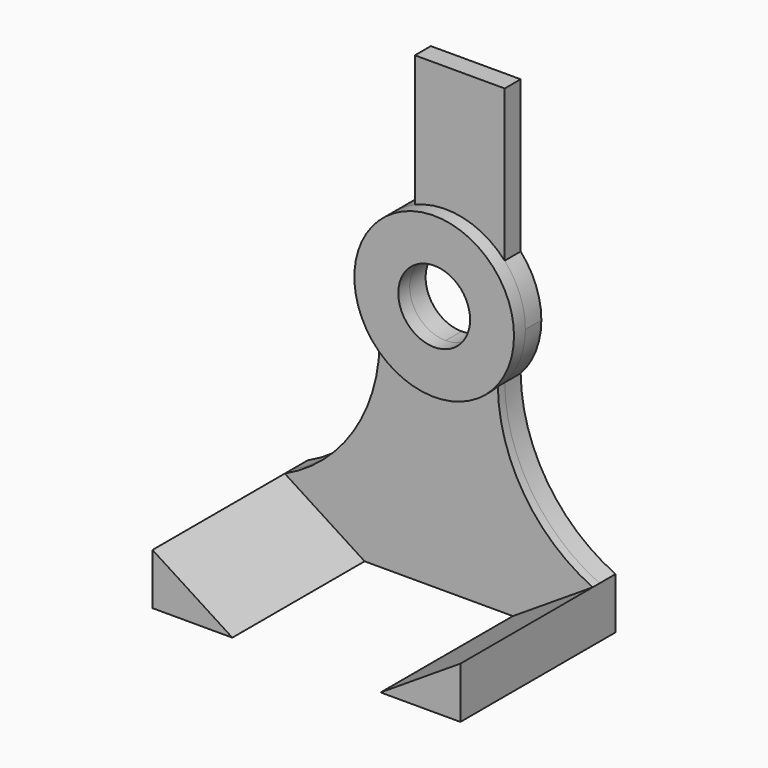
from build123d import *
from build123d import SkipClean  # not in build123d's __all__

# Parameters (mm, degrees)
F1_DEPTH = 5.55625
F2_R     = 22.225
F2_R_2   = 10.0000054
F3_DEPTH = 3.96875
F5_DEPTH = 2.38125
F7_DEPTH = 46.0375


# Not quite as in the source:
# - after a boolean that leaves OpenCascade's solid faulty, fix() repairs it


with BuildPart() as f1:
    # F0 (on Front) → F1 (new body)
    with BuildSketch(Plane.XZ):
        with BuildLine():
            ThreePointArc((8.5411146283, 90.3682841852), (21.9263912189, 91.5406597383), (33.5411154283, 84.7850490788))
            Line((33.5411154283, 84.7850490788), (33.5411154283, 127))
            Line((33.5411154283, 127), (8.5411146283, 127))
            Line((8.5411146283, 127), (8.5411146283, 90.3682841852))
        make_face()
        with BuildLine():
            ThreePointArc((17.0822292566, 47.625), (26.0827614415, 49.5290491023), (33.5411154283, 54.9149509212))
            Line((33.5411154283, 54.9149509212), (33.5411154283, 84.7850490788))
            ThreePointArc((33.5411154283, 84.7850490788), (21.9263912189, 91.5406597383), (8.5411146283, 90.3682841852))
            Line((8.5411146283, 90.3682841852), (8.5411146283, 75.050910392))
            ThreePointArc((8.5411146283, 75.050910392), (19.7830546485, 79.4783773401), (27.0822346566, 69.85))
            ThreePointArc((27.0822346566, 69.85), (24.1533008869, 62.7789283698), (17.0822292566, 59.8499946))
            Line((17.0822292566, 59.8499946), (17.0822292566, 47.625))
        make_face()
        with BuildLine():
            ThreePointArc((0.6233430849, 54.9149509212), (8.0816970717, 49.5290491023), (17.0822292566, 47.625))
            Line((17.0822292566, 47.625), (17.0822292566, 59.8499946))
            ThreePointArc((17.0822292566, 59.8499946), (8.3641663982, 64.9514810404), (8.5411146283, 75.050910392))
            Line((8.5411146283, 75.050910392), (8.5411146283, 90.3682841852))
            ThreePointArc((8.5411146283, 90.3682841852), (-4.6084304817, 74.6941619623), (0.6233430849, 54.9149509212))
        make_face()
        with BuildLine():
            Line((33.5411154283, 84.7850490788), (33.5411154283, 54.9149509212))
            ThreePointArc((33.5411154283, 54.9149509212), (37.8156487788, 61.8452551623), (39.3072292566, 69.85))
            ThreePointArc((39.3072292566, 69.85), (37.8156487788, 77.8547448377), (33.5411154283, 84.7850490788))
        make_face()
        with BuildLine():
            Line((17.0822292566, 0), (17.0822292566, 47.625))
            ThreePointArc((17.0822292566, 47.625), (8.0816970717, 49.5290491023), (0.6233430849, 54.9149509212))
            ThreePointArc((0.6233430849, 54.9149509212), (-6.7205760102, 30.7942081775), (-25.7802707434, 14.2875))
            Line((-25.7802707434, 14.2875), (-25.7802707434, 0))
            Line((-25.7802707434, 0), (17.0822292566, 0))
        make_face()
        with BuildLine():
            Line((33.5411154283, 0), (33.5411154283, 54.9149509212))
            ThreePointArc((33.5411154283, 54.9149509212), (26.0827614415, 49.5290491023), (17.0822292566, 47.625))
            Line((17.0822292566, 47.625), (17.0822292566, 0))
            Line((17.0822292566, 0), (33.5411154283, 0))
        make_face()
        with BuildLine():
            ThreePointArc((59.9447292566, 14.2875), (40.8850345234, 30.7942081775), (33.5411154283, 54.9149509212))
            Line((33.5411154283, 54.9149509212), (33.5411154283, 0))
            Line((33.5411154283, 0), (59.9447292566, 0))
            Line((59.9447292566, 0), (59.9447292566, 14.2875))
        make_face()
    extrude(amount=F1_DEPTH)

    # F2 (on face) → F3 (join)
    with BuildSketch(Plane.XZ.offset(5.55625)):
        with Locations((17.0822292566, 69.85)):
            Circle(F2_R)
        with Locations((17.0822292566, 69.85)):
            Circle(F2_R_2, mode=Mode.SUBTRACT)
    with SkipClean():  # cleaning this boolean's faces spoils the solid; the shape is the same uncleaned
        extrude(amount=F3_DEPTH)

    # F3_face (on face) + F4 (on face) → F5 (join)
    with BuildSketch(Plane(origin=(17.0822292566, -5.55625, 20.2916476737), x_dir=(1, 0, 0), z_dir=(0, -1, 0))):
        with BuildLine():
            ThreePointArc((16.4588861717, 34.6233032475), (0, 27.3333523263), (-16.4588861717, 34.6233032475))
            ThreePointArc((-16.4588861717, 34.6233032475), (-23.8028052668, 10.5025605039), (-42.8625, -6.0041476737))
            Line((-42.8625, -6.0041476737), (-42.8625, -20.2916476737))
            Line((-42.8625, -20.2916476737), (42.8625, -20.2916476737))
            Line((42.8625, -20.2916476737), (42.8625, -6.0041476737))
            ThreePointArc((42.8625, -6.0041476737), (23.8028052668, 10.5025605039), (16.4588861717, 34.6233032475))
        make_face()
    with BuildSketch(Plane.XZ.offset(5.55625)):
        with BuildLine():
            ThreePointArc((59.9447292566, 14.2875), (40.8850345234, 30.7942081775), (33.5411154283, 54.9149509212))
            ThreePointArc((33.5411154283, 54.9149509212), (17.0822292566, 47.625), (0.6233430849, 54.9149509212))
            ThreePointArc((0.6233430849, 54.9149509212), (-6.7205760102, 30.7942081775), (-25.7802707434, 14.2875))
            Line((-25.7802707434, 14.2875), (-25.7802707434, 0))
            Line((-25.7802707434, 0), (59.9447292566, 0))
            Line((59.9447292566, 0), (59.9447292566, 14.2875))
        make_face()
    extrude(amount=F5_DEPTH)

    add(f1.part.fix(), mode=Mode.REPLACE)

    # F6 (on face) → F7 (join)
    with BuildSketch(Plane.XZ.offset(7.9375)):
        Polygon((-25.7802707434, 14.2875), (-25.7802707434, 0), (-3.5552707434, 0), align=None)
        Polygon((59.9447292566, 14.2875), (37.7197292566, 0), (59.9447292566, 0), align=None)
    extrude(amount=F7_DEPTH)


solid = f1.part
